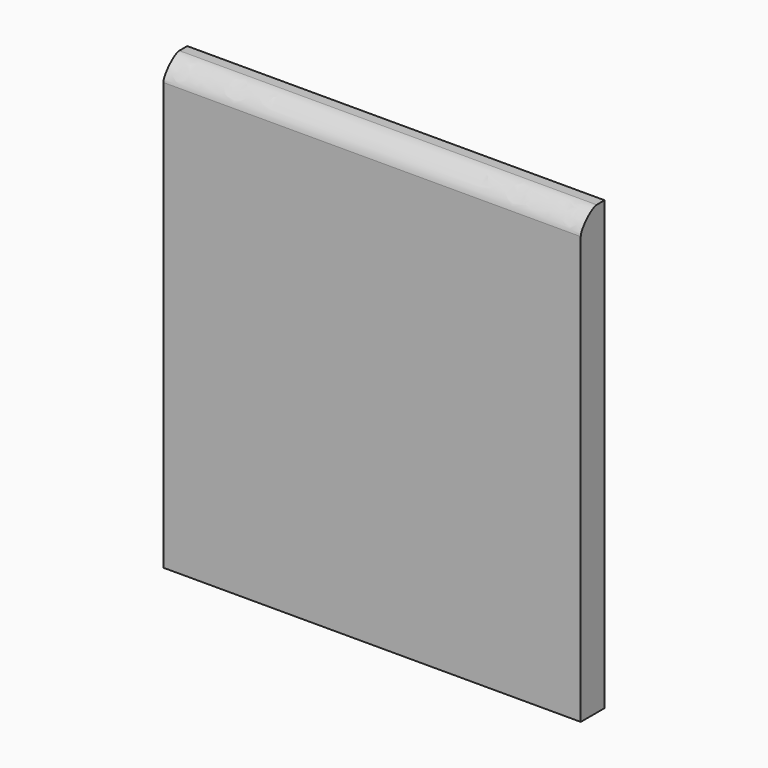
from build123d import *

# Parameters (mm, degrees)
F0_W        = 12.7
F0_H        = 76.2
F0_H_2      = 57.15
F1_DEPTH    = 19.05
F2_T1_DEPTH = 330.2


# Not quite as in the source:
# - a fillet or chamfer that OpenCascade refuses, or shapes differently, is made with other operations: its cross-section is extruded or revolved along the edge and cut away or added


with BuildPart() as f1:
    # F0 (on Front) → F1 (new body)
    with BuildSketch(Plane.XZ):
        Polygon((-266.7, 0), (0, 0), (0, 209.55), (-254, 209.55), (-266.7, 209.55), align=None)
        with Locations((-260.35, 247.65)):
            Rectangle(F0_W, F0_H)
        with Locations((-6.35, 257.175)):
            Rectangle(F0_W, F0_H_2)
        Polygon((-254, 209.55), (0, 209.55), (0, 228.6), (-12.7, 228.6), (-12.7, 285.75), (-254, 285.75), align=None)
    extrude(amount=F1_DEPTH)

    # F2: fillet of radius 12.7 on 1 edges, made by hand

    # F2_s2 → F2_t1 (cut)
    with BuildSketch(Plane.YZ.offset(-298.45)):
        with BuildLine():
            add(Edge.make_bspline(
                [(-6.35, 285.75), (-19.05, 285.75), (-19.05, 273.05)],
                knots=[0, 0, 0, 1, 1, 1], degree=2, weights=[1, 0.3333333333, 1]))
            Line((-19.05, 273.05), (-19.05, 285.75))
            Line((-19.05, 285.75), (-6.35, 285.75))
        make_face()
    extrude(amount=F2_T1_DEPTH, mode=Mode.SUBTRACT)


solid = f1.part
